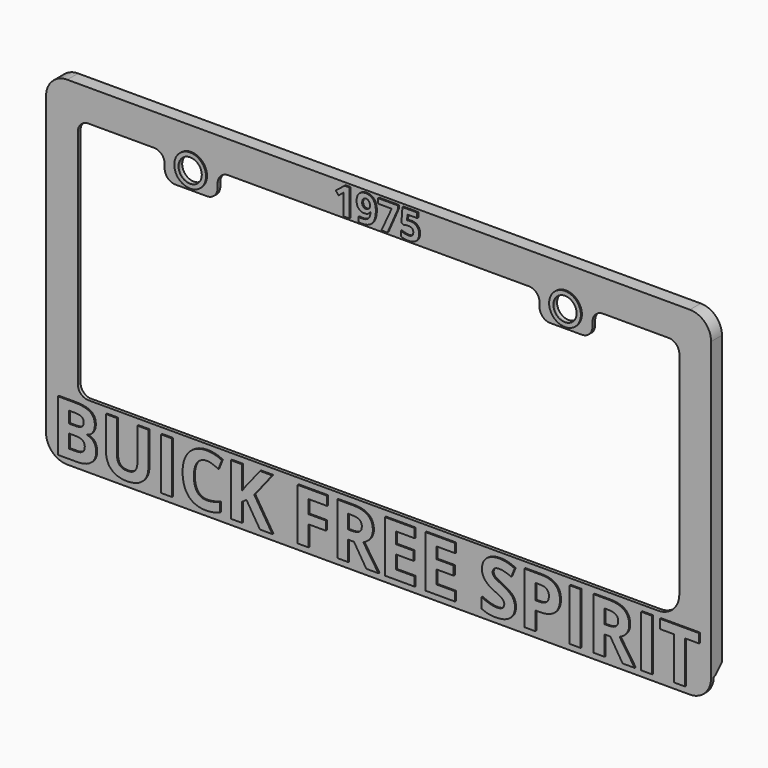
from build123d import *

# Parameters (mm, degrees)
F1_DEPTH      = 1.6
F2_W          = 25
F2_H          = 12
F3_DEPTH      = 1.6
F5_R          = 5
F6_R          = 5.5
F7_DEPTH      = 25
F8_TEXT_SIZE  = 18.0555555556
F9_DEPTH      = 0.6
F11_TEXT_SIZE = 34.0937786464
F12_DEPTH     = 0.6
F14_DEPTH     = 4.8
F16_DEPTH     = 1.6
F17_SIZE      = 4.2
F18_R         = 7.5
F18_R_2       = 5.5
F19_DEPTH     = 0.6


# Not quite as in the source:
# - Text() gives the source's letters only with a copy of the font that has no kerning and outlines rounded to 1/6400 em; it was checked with that copy


with BuildPart() as f1:
    # F0 (on Front) → F1 (new body)
    with BuildSketch(Plane.XZ):
        with BuildLine():
            ThreePointArc((157, 70), (154.0710678119, 77.0710678119), (147, 80))
            Line((147, 80), (-147, 80))
            ThreePointArc((-147, 80), (-154.0710678119, 77.0710678119), (-157, 70))
            Line((-157, 70), (-157, -70))
            ThreePointArc((-157, -70), (-154.0710678119, -77.0710678119), (-147, -80))
            Line((-147, -80), (147, -80))
            ThreePointArc((147, -80), (154.0710678119, -77.0710678119), (157, -70))
            Line((157, -70), (157, 70))
        make_face()
        with BuildLine():
            Line((-137, 65), (137, 65))
            ThreePointArc((137, 65), (140.5355339059, 63.5355339059), (142, 60))
            Line((142, 60), (142, -40))
            ThreePointArc((142, -40), (139.0710678119, -47.0710678119), (132, -50))
            Line((132, -50), (-137, -50))
            ThreePointArc((-137, -50), (-140.5355339059, -48.5355339059), (-142, -45))
            Line((-142, -45), (-142, 60))
            ThreePointArc((-142, 60), (-140.5355339059, 63.5355339059), (-137, 65))
        make_face(mode=Mode.SUBTRACT)
    extrude(amount=F1_DEPTH)

    # F2 (on face) → F3 (join, through all)
    with BuildSketch(Plane.XZ.offset(1.6)):
        with Locations((-88.5, 59)):
            Rectangle(F2_W, F2_H)
        with Locations((88.5, 59)):
            Rectangle(F2_W, F2_H)
    extrude(amount=-F3_DEPTH)

    # F5
    f5_edges = [f1.edges().sort_by_distance(p)[0] for p in [
        (-101, -0.8, 53),
        (-101, -0.8, 65),
        (-76, -0.8, 53),
        (-76, -0.8, 65),
        (101, -0.8, 53),
        (101, -0.8, 65),
        (76, -0.8, 53),
        (76, -0.8, 65),
    ]]
    fillet(f5_edges, radius=F5_R)

    # F6 (on face) → F7 (cut)
    with BuildSketch(Plane.XZ.offset(1.6)):
        with Locations((-88.5, 61.5)):
            Circle(F6_R)
        with Locations((88.5, 61.5)):
            Circle(F6_R)
    extrude(amount=-F7_DEPTH, mode=Mode.SUBTRACT)

    # F8 (on face) → F9 (join)
    with BuildSketch(Plane.XZ.offset(1.6)):
        with Locations((-20.7921006944, 66)):
            Text('1975', F8_TEXT_SIZE, font='Open Sans', font_style=FontStyle.BOLD, text_align=(TextAlign.LEFT, TextAlign.BOTTOM))
    extrude(amount=F9_DEPTH)

    # F11 (on face) → F12 (join)
    with BuildSketch(Plane.XZ.offset(1.6)):
        with Locations((-154, -77)):
            Text('BUICK FREE SPIRIT', F11_TEXT_SIZE, font='Open Sans', font_style=FontStyle.BOLD, text_align=(TextAlign.LEFT, TextAlign.BOTTOM))
    extrude(amount=F12_DEPTH)

    # F13 (on face) → F14 (join)
    with BuildSketch(Plane(origin=(0, 0, 0), x_dir=(-1, 0, 0), z_dir=(0, 1, 0))):
        with BuildLine():
            ThreePointArc((-147, 80), (-154.0710678119, 77.0710678119), (-157, 70))
            Line((-157, 70), (-157, -70))
            Line((-157, -70), (-155, -70))
            Line((-155, -70), (-155, 70))
            ThreePointArc((-155, 70), (-152.6568542495, 75.6568542495), (-147, 78))
            Line((-147, 78), (147, 78))
            ThreePointArc((147, 78), (152.6568542495, 75.6568542495), (155, 70))
            Line((155, 70), (155, -70))
            Line((155, -70), (157, -70))
            Line((157, -70), (157, 70))
            ThreePointArc((157, 70), (154.0710678119, 77.0710678119), (147, 80))
            Line((147, 80), (-147, 80))
        make_face()
    extrude(amount=F14_DEPTH)

    # F15 (on face) → F16 (join)
    with BuildSketch(Plane(origin=(0, 4.8, 0), x_dir=(-1, 0, 0), z_dir=(0, 1, 0))):
        Polygon((-155, 31), (-155, -31), (-150, -31), (-150, 25.041232037), align=None)
        Polygon((150, -31), (155, -31), (155, 31), (150, 25.041232037), align=None)
    extrude(amount=-F16_DEPTH)

    # F17
    f17_edges = [f1.edges().sort_by_distance(p)[0] for p in [
        (-156, 4.8, -70),
        (156, 4.8, -70),
    ]]
    chamfer(f17_edges, length=F17_SIZE)

    # F18 (on face) → F19 (join)
    with BuildSketch(Plane.XZ.offset(1.6)):
        with Locations((-88.5, 61.5)):
            Circle(F18_R)
        with Locations((-88.5, 61.5)):
            Circle(F18_R_2, mode=Mode.SUBTRACT)
        with Locations((88.5, 61.5)):
            Circle(F18_R)
        with Locations((88.5, 61.5)):
            Circle(F18_R_2, mode=Mode.SUBTRACT)
    extrude(amount=F19_DEPTH)


solid = f1.part
